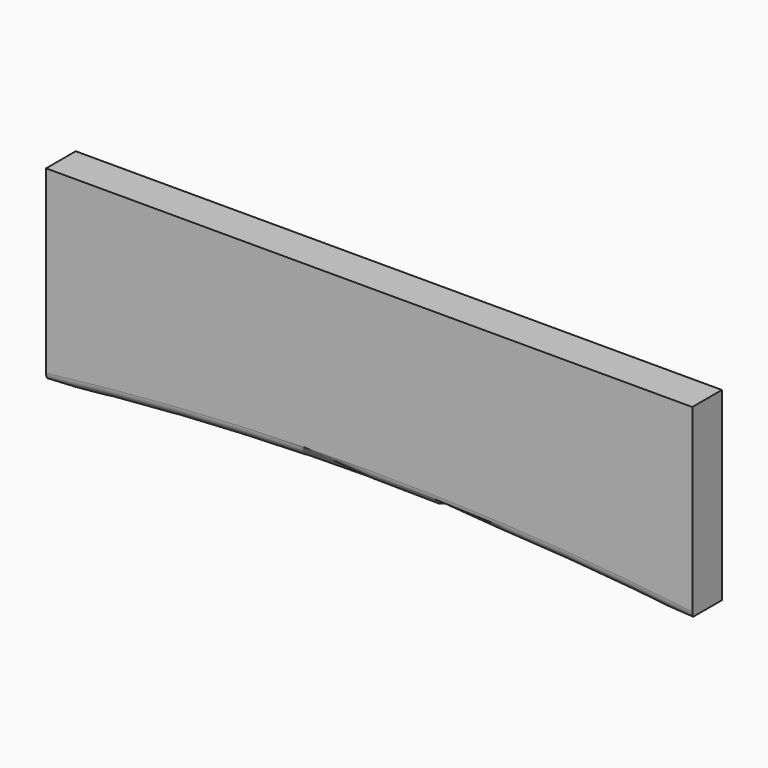
from build123d import *

# Parameters (mm, degrees)
F1_DEPTH    = 17.4625
F2_T2_ANGLE = 17.1649477786


# Not quite as in the source:
# - a fillet or chamfer that OpenCascade refuses, or shapes differently, is made with other operations: its cross-section is extruded or revolved along the edge and cut away or added


with BuildPart() as f1:
    # F0 (on Front) → F1 (new body)
    with BuildSketch(Plane.XZ):
        with BuildLine():
            Line((0, 87.3125), (0, 0))
            Line((0, 0), (25.4, 0))
            ThreePointArc((25.4, 0), (152.4, 6.35), (279.4, 0))
            Line((279.4, 0), (304.8, 0))
            Line((304.8, 0), (304.8, 87.3125))
            Line((304.8, 87.3125), (0, 87.3125))
        make_face()
    extrude(amount=F1_DEPTH)

    # F2: fillet of radius 5.08 on 1 edges, made by hand

    # F2_s1 → F2_t2 (revolve, cut)
    with BuildSketch(Plane(origin=(-37.9289804695, 0, -5.7243521326), x_dir=(0, 1, 0), z_dir=(-0.9888020759, 0, -0.1492328874))):
        with BuildLine():
            ThreePointArc((-12.3825, 2.2072818505), (-15.9746024484, 0.7193842989), (-17.4625, -2.8727181495))
            Line((-17.4625, -2.8727181495), (-17.4625, 2.2072818505))
            Line((-17.4625, 2.2072818505), (-12.3825, 2.2072818505))
        make_face()
    revolve(axis=Axis((152.4, -17.4625, -1266.8250000001), (0, 1, 0)), revolution_arc=F2_T2_ANGLE, mode=Mode.SUBTRACT)


solid = f1.part
